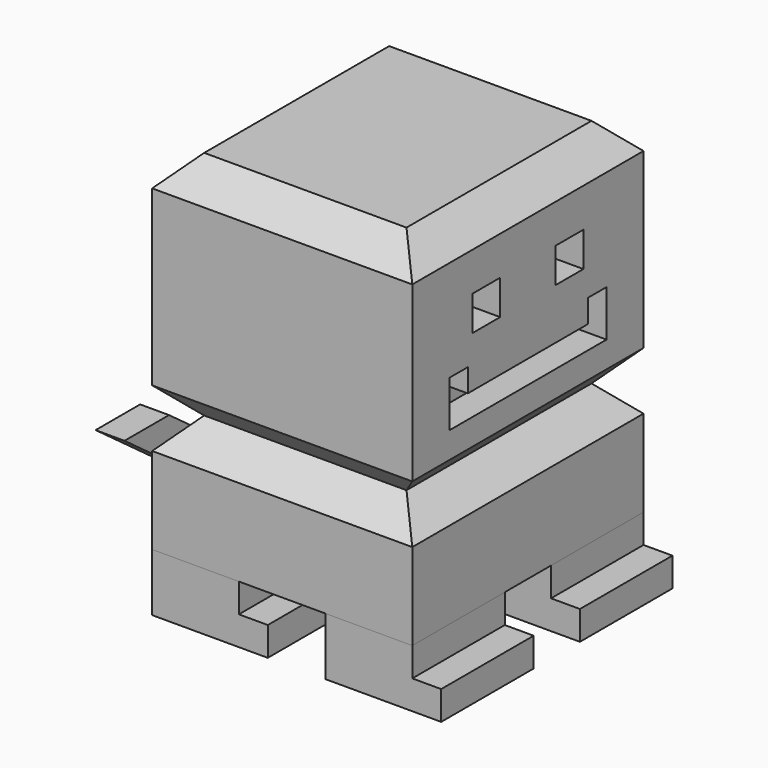
from build123d import *

# Parameters (mm, degrees)
F0_W      = 20
F0_H      = 20
F1_DEPTH  = 10
F2_W      = 5
F2_H      = 20
F3_DEPTH  = 5
F4_W      = 15
F4_H      = 20
F5_DEPTH  = 20
F6_SIZE   = 5
F7_W      = 45
F7_H      = 50
F7_W_2    = 35
F7_H_2    = 40
F8_DEPTH  = 40
F9_SIZE   = 4.99999
F10_SIZE  = 5
F11_W     = 6
F11_H     = 6
F11_W_2   = 26
F11_H_2   = 4
F12_DEPTH = 5
F14_W     = 9.7873052548
F14_H     = 10
F14_H_2   = 20
F16_DEPTH = 15
F18_W     = 4.7873052548
F18_H     = 10
F19_DEPTH = 30
F20_DEPTH = 9.7873052548


# Not quite as in the source:
# - a fillet or chamfer is up to 0.001 mm smaller than in the source, because OpenCascade refuses the exact size


with BuildPart() as f1:
    # F0 (on Top) → F1 (new body)
    with BuildSketch(Plane.XY):
        with Locations((19.7873052548, -35.1500818506)):
            Rectangle(F0_W, F0_H)
    extrude(amount=F1_DEPTH)


with BuildPart() as f1b:
    # F0 (on Top) → F1, piece 2 (new body)
    with BuildSketch(Plane.XY):
        with Locations((19.7873052548, -5.1500818506)):
            Rectangle(F0_W, F0_H)
    extrude(amount=F1_DEPTH)


with BuildPart() as f1c:
    # F0 (on Top) → F1, piece 3 (new body)
    with BuildSketch(Plane.XY):
        with Locations((49.7873052548, -35.1500818506)):
            Rectangle(F0_W, F0_H)
    extrude(amount=F1_DEPTH)


with BuildPart() as f1d:
    # F0 (on Top) → F1, piece 4 (new body)
    with BuildSketch(Plane.XY):
        with Locations((49.7873052548, -5.1500818506)):
            Rectangle(F0_W, F0_H)
    extrude(amount=F1_DEPTH)


with BuildPart() as f3_tool:
    # F2 (on face) → F3 (new body)
    with BuildSketch(Plane.XY.offset(10)):
        with Locations((57.2873052548, -35.1500818506)):
            Rectangle(F2_W, F2_H)
        with Locations((57.2873052548, -5.1500818506)):
            Rectangle(F2_W, F2_H)
        with Locations((27.2873052548, -35.1500818506)):
            Rectangle(F2_W, F2_H)
        with Locations((27.2873052548, -5.1500818506)):
            Rectangle(F2_W, F2_H)
    extrude(amount=-F3_DEPTH)


with BuildPart() as f1_1:
    add(f1.part)

    # F3: cut by f3_tool
    add(f3_tool.part, mode=Mode.SUBTRACT)


with BuildPart() as f1b_1:
    add(f1b.part)

    # F3: cut by f3_tool
    add(f3_tool.part, mode=Mode.SUBTRACT)


with BuildPart() as f1c_1:
    add(f1c.part)

    # F3: cut by f3_tool
    add(f3_tool.part, mode=Mode.SUBTRACT)


with BuildPart() as f1d_1:
    add(f1d.part)

    # F3: cut by f3_tool
    add(f3_tool.part, mode=Mode.SUBTRACT)


with BuildPart() as f5:
    # F4 (on face) → F5 (new body)
    with BuildSketch(Plane.XY.offset(10)):
        Polygon((54.7873052548, 4.8499181494), (24.7873052548, 4.8499181494), (24.7873052548, -15.1500818506), (9.7873052548, -15.1500818506), (9.7873052548, -45.1500818506), (54.7873052548, -45.1500818506), align=None)
        with Locations((17.2873052548, -5.1500818506)):
            Rectangle(F4_W, F4_H)
    extrude(amount=F5_DEPTH)

    # F6
    f6_edges = [f5.edges().sort_by_distance(p)[0] for p in [
        (32.287305, 4.849918, 30),
        (54.787305, -20.150082, 30),
        (32.287305, -45.150082, 30),
        (9.787305, -20.150082, 30),
    ]]
    chamfer(f6_edges, length=F6_SIZE)

    # F7 (on face) → F8 (join)
    with BuildSketch(Plane.XY.offset(30)):
        with Locations((32.2873052548, -20.1500818506)):
            Rectangle(F7_W, F7_H)
        with Locations((32.2873052548, -20.1500818506)):
            Rectangle(F7_W_2, F7_H_2, mode=Mode.SUBTRACT)
        with Locations((32.2873052548, -20.1500818506)):
            Rectangle(F7_W_2, F7_H_2)
    extrude(amount=F8_DEPTH)

    # F9 (size 5 in the source; OpenCascade refuses exactly that, so slightly less here)
    f9_edges = [f5.edges().sort_by_distance(p)[0] for p in [
        (32.287305, -45.150082, 30),
        (54.787305, -20.150082, 30),
        (32.287305, 4.849918, 30),
        (9.787305, -20.150082, 30),
    ]]
    chamfer(f9_edges, length=F9_SIZE)

    # F10
    f10_edges = [f5.edges().sort_by_distance(p)[0] for p in [
        (32.287305, -45.150082, 70),
        (54.787305, -20.150082, 70),
        (32.287305, 4.849918, 70),
        (9.787305, -20.150082, 70),
    ]]
    chamfer(f10_edges, length=F10_SIZE)

    # F11 (on face) → F12 (cut)
    with BuildSketch(Plane.YZ.offset(54.7873052548)):
        with Locations((-29.1500818506, 55.3023344576)):
            Rectangle(F11_W, F11_H)
        with Locations((-11.1500818506, 55.3023344576)):
            Rectangle(F11_W, F11_H)
        Polygon((-33.1500818506, 47.5259826481), (-37.1500818506, 47.5259826481), (-37.1500818506, 39.5259826481), (-33.1500818506, 39.5259826481), (-33.1500818506, 43.5259826481), align=None)
        with Locations((-20.1500818506, 41.5259826481)):
            Rectangle(F11_W_2, F11_H_2)
        Polygon((-7.1500818506, 47.5259826481), (-7.1500818506, 43.5259826481), (-7.1500818506, 39.5259826481), (-3.1500818506, 39.5259826481), (-3.1500818506, 47.5259826481), align=None)
    extrude(amount=-F12_DEPTH, mode=Mode.SUBTRACT)

    # F14 (on offset) → F16 (join)
    with BuildSketch(Plane.XY.offset(10)):
        with Locations((4.8936526274, -20.1500818506)):
            Rectangle(F14_W, F14_H)
        with Locations((4.8936526274, -35.1500818506)):
            Rectangle(F14_W, F14_H_2)
    extrude(amount=F16_DEPTH)

    # F18 (on face) → F19 (cut, through all)
    with BuildSketch(Plane.XZ.offset(45.1500818506)):
        with Locations((7.3936526274, 20)):
            Rectangle(F18_W, F18_H)
    extrude(amount=-F19_DEPTH, mode=Mode.SUBTRACT)

    # F17 (on face) → F20 (cut, through all)
    with BuildSketch(Plane(origin=(0, 0, 0), x_dir=(0, -1, 0), z_dir=(-1, 0, 0))):
        Polygon((15.1500818506, 25), (15.1500818506, 10), (35.5198492855, 25), align=None)
        Polygon((45.1500818506, 25), (24.7803144157, 10), (45.1500818506, 10), align=None)
    extrude(amount=-F20_DEPTH, mode=Mode.SUBTRACT)


solid = Compound([f1_1.part, f1b_1.part, f1c_1.part, f1d_1.part, f5.part])
